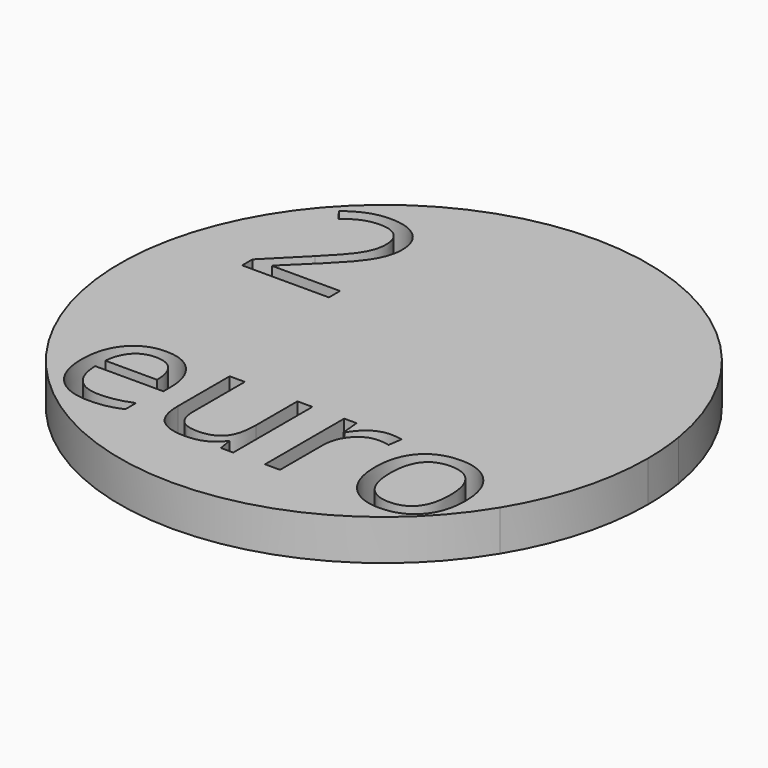
from build123d import *

# Parameters (mm, degrees)
F1_DEPTH     = 2
F2_TEXT_SIZE = 9.1083754359
F3_DEPTH     = 2.001


# Not quite as in the source:
# - Text() gives the source's letters only with a copy of the font that has no kerning and outlines rounded to 1/6400 em; it was checked with that copy


with BuildPart() as f1:
    # F0 (on Top) → F1 (new body)
    with BuildSketch(Plane.XY):
        with BuildLine():
            ThreePointArc((51.0762404, 10.8613331262), (51.0339172206, 11.9094797825), (50.9072232595, 12.9508016851))
            ThreePointArc((50.9072232595, 12.9508016851), (48.9736524431, 8.739268037), (49.1856304111, 4.1099293031))
            ThreePointArc((49.1856304111, 4.1099293031), (50.5946682195, 7.3557711273), (51.0762404, 10.8613331262))
        make_face()
        with BuildLine():
            ThreePointArc((49.1856304111, 4.1099293031), (48.9736524431, 8.739268037), (50.9072232595, 12.9508016851))
            ThreePointArc((50.9072232595, 12.9508016851), (41.6140324577, 23.3706907178), (28.2400826135, 19.3613331262))
            Line((28.2400826135, 19.3613331262), (33.0990423931, 19.3613331262))
            ThreePointArc((33.0990423931, 19.3613331262), (42.9750718745, 19.4067383351), (47.9262404, 10.8613331262))
            ThreePointArc((47.9262404, 10.8613331262), (42.9750718745, 2.3159279173), (33.0990423931, 2.3613331262))
            Line((33.0990423931, 2.3613331262), (28.2400826135, 2.3613331262))
            ThreePointArc((28.2400826135, 2.3613331262), (39.1577565682, -2.0936011762), (49.1856304111, 4.1099293031))
        make_face()
        with BuildLine():
            Line((33.0990423931, 19.3613331262), (28.2400826135, 19.3613331262))
            ThreePointArc((28.2400826135, 19.3613331262), (25.0762404, 10.8613331262), (28.2400826135, 2.3613331262))
            Line((28.2400826135, 2.3613331262), (33.0990423931, 2.3613331262))
            ThreePointArc((33.0990423931, 2.3613331262), (28.2262404, 10.8613331262), (33.0990423931, 19.3613331262))
        make_face()
        with BuildLine():
            Line((38.0762404, 19.3613331262), (33.0990423931, 19.3613331262))
            ThreePointArc((33.0990423931, 19.3613331262), (28.2262404, 10.8613331262), (33.0990423931, 2.3613331262))
            Line((33.0990423931, 2.3613331262), (38.0762404, 2.3613331262))
            ThreePointArc((38.0762404, 2.3613331262), (29.5762404, 10.8613331262), (38.0762404, 19.3613331262))
        make_face()
        with BuildLine():
            ThreePointArc((46.5762404, 10.8613331262), (44.0866480401, 16.8717407663), (38.0762404, 19.3613331262))
            ThreePointArc((38.0762404, 19.3613331262), (29.5762404, 10.8613331262), (38.0762404, 2.3613331262))
            ThreePointArc((38.0762404, 2.3613331262), (44.0866480401, 4.8509254861), (46.5762404, 10.8613331262))
        make_face()
        with BuildLine():
            ThreePointArc((47.9262404, 10.8613331262), (42.9750718745, 19.4067383351), (33.0990423931, 19.3613331262))
            Line((33.0990423931, 19.3613331262), (38.0762404, 19.3613331262))
            ThreePointArc((38.0762404, 19.3613331262), (44.0866480401, 16.8717407663), (46.5762404, 10.8613331262))
            ThreePointArc((46.5762404, 10.8613331262), (44.0866480401, 4.8509254861), (38.0762404, 2.3613331262))
            Line((38.0762404, 2.3613331262), (33.0990423931, 2.3613331262))
            ThreePointArc((33.0990423931, 2.3613331262), (42.9750718745, 2.3159279173), (47.9262404, 10.8613331262))
        make_face()
    extrude(amount=F1_DEPTH)

    # F2 (on face) → F3 (cut, through all)
    with BuildSketch(Plane.XY.offset(2)):
        with Locations((28.400702365, 13.6715878564)):
            Text('2', F2_TEXT_SIZE, font='Open Sans', text_align=(TextAlign.LEFT, TextAlign.BOTTOM))
        with Locations((28.400702365, 1.2841972637)):
            Text('euro', F2_TEXT_SIZE, font='Open Sans', text_align=(TextAlign.LEFT, TextAlign.BOTTOM))
    extrude(amount=-F3_DEPTH, mode=Mode.SUBTRACT)


solid = f1.part
